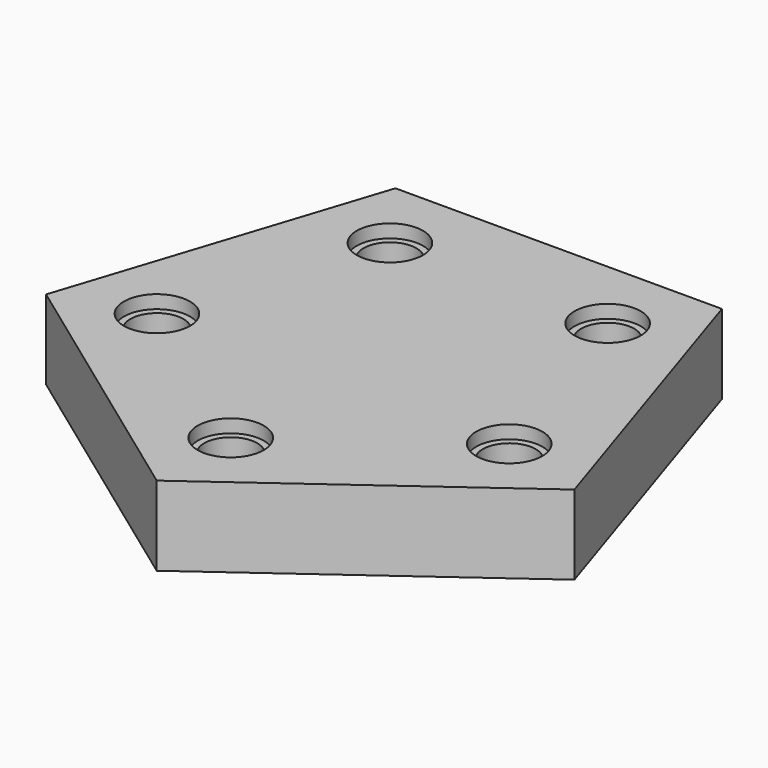
from build123d import *

# Parameters (mm, degrees)
F0_R     = 1
F1_DEPTH = 3
F2_R     = 1.25
F3_DEPTH = 0.5


# Not quite as in the source:
# - a pattern or mirror of a feature is missing from the dataset's text; its kind, count and spacing are read off the source's solid


with BuildPart() as f1:
    # F0 (on Top) → F1 (new body)
    with BuildSketch(Plane.XY):
        Polygon((6.17, 8.4922764493), (-6.17, 8.4922764493), (-9.9832697106, -3.2437609618), (0, -10.4970309751), (9.9832697106, -3.2437609618), align=None)
        with Locations((-6.6573956141, -2.1631189606)):
            Circle(F0_R, mode=Mode.SUBTRACT)
        with Locations((0, -7)):
            Circle(F0_R, mode=Mode.SUBTRACT)
        with Locations((6.6573956141, -2.1631189606)):
            Circle(F0_R, mode=Mode.SUBTRACT)
        with Locations((-4.114496766, 5.6631189606)):
            Circle(F0_R, mode=Mode.SUBTRACT)
        with Locations((4.114496766, 5.6631189606)):
            Circle(F0_R, mode=Mode.SUBTRACT)
    extrude(amount=F1_DEPTH)

    # F2 (on face) → F3 (cut)
    with BuildSketch(Plane.XY.offset(3)):
        with Locations((0, -7)):
            Circle(F2_R)
        with Locations((6.6573956141, -2.1631189606)):
            Circle(F2_R)
        with Locations((4.114496766, 5.6631189606)):
            Circle(F2_R)
        with Locations((-4.114496766, 5.6631189606)):
            Circle(F2_R)
        with Locations((-6.6573956141, -2.1631189606)):
            Circle(F2_R)
    f3 = extrude(amount=-F3_DEPTH, mode=Mode.SUBTRACT)

    # F3_copies: F3 across plane
    add(f3.mirror(Plane(origin=(0, 0, 1.5), x_dir=(-1, 0, 0), z_dir=(0, 0, -1))), mode=Mode.SUBTRACT)


solid = f1.part
